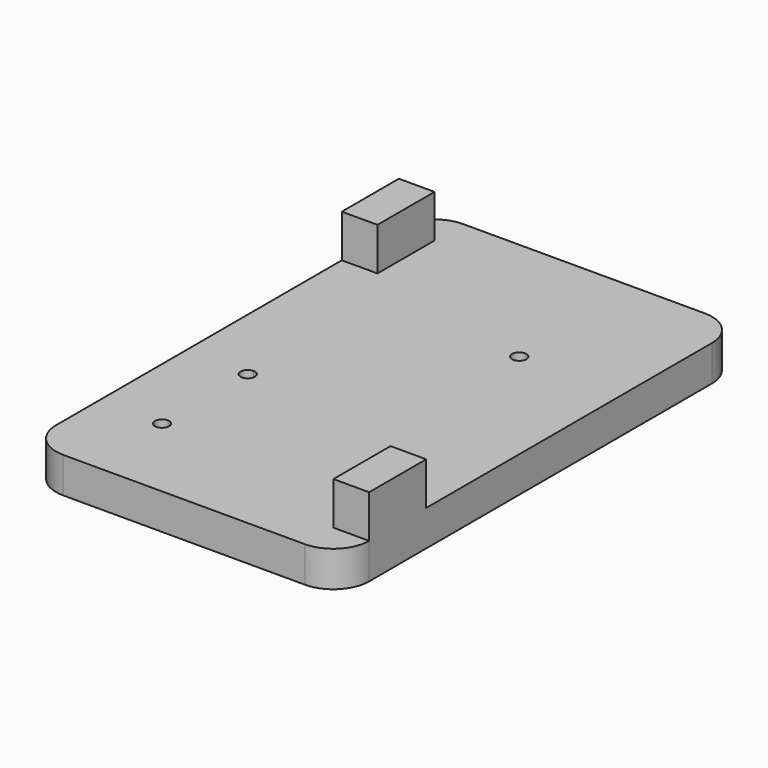
from build123d import *

# Parameters (mm, degrees)
F1_DEPTH = 5
F2_W     = 10
F2_H     = 5
F3_DEPTH = 6
F2_W_2   = 5
F2_H_2   = 10


with BuildPart() as f1:
    # F0 (on Top) → F1 (new body)
    with BuildSketch(Plane.XY):
        with BuildLine():
            ThreePointArc((0, 5), (1.4644660941, 1.4644660941), (5, 0))
            Line((5, 0), (38.87, 0))
            ThreePointArc((38.87, 0), (42.4055339059, 1.4644660941), (43.87, 5))
            Line((43.87, 5), (43.87, 49.36))
            Line((43.87, 49.36), (43.87, 65.05))
            ThreePointArc((43.87, 65.05), (42.4055339059, 68.5855339059), (38.87, 70.05))
            Line((38.87, 70.05), (5, 70.05))
            ThreePointArc((5, 70.05), (1.4644660941, 68.5855339059), (0, 65.05))
            Line((0, 65.05), (0, 5))
        make_face()
        with BuildLine():
            ThreePointArc((9.82, 12.55), (8.1128932188, 11.8428932188), (8.82, 13.55))
            ThreePointArc((8.82, 13.55), (9.5271067812, 13.2571067812), (9.82, 12.55))
        make_face(mode=Mode.SUBTRACT)
        with BuildLine():
            ThreePointArc((8.82, 26.55), (7.82, 27.55), (8.82, 28.55))
            ThreePointArc((8.82, 28.55), (9.5271067812, 28.2571067812), (9.82, 27.55))
            ThreePointArc((9.82, 27.55), (9.5271067812, 26.8428932188), (8.82, 26.55))
        make_face(mode=Mode.SUBTRACT)
        with BuildLine():
            ThreePointArc((28.42, 49.36), (29.42, 50.36), (30.42, 49.36))
            ThreePointArc((30.42, 49.36), (29.42, 48.36), (28.42, 49.36))
        make_face(mode=Mode.SUBTRACT)
    extrude(amount=F1_DEPTH)

    # F2 (on face) → F3, piece 2 (join)
    with BuildSketch(Plane.XY.offset(5)):
        with Locations((41.37, 10)):
            Rectangle(F2_W_2, F2_H_2)
        with Locations((2.5, 60.05)):
            Rectangle(F2_W_2, F2_H_2)
    extrude(amount=F3_DEPTH)


with BuildPart() as f3:
    # F2 (on face) → F3 (new body)
    with BuildSketch(Plane.XY.offset(5)):
        with Locations((33.87, 2.5)):
            Rectangle(F2_W, F2_H)
    extrude(amount=F3_DEPTH)


solid = f1.part
